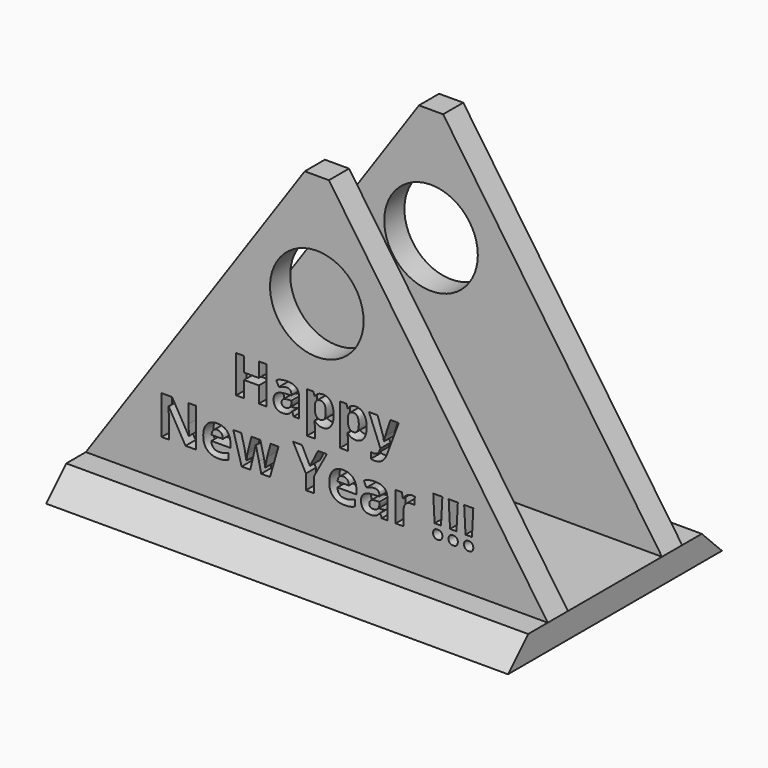
from build123d import *

# Parameters (mm, degrees)
F0_W            = 55
F0_H            = 14
F1_DEPTH        = 3
F2_W            = 55
F2_H            = 3
F3_DEPTH        = 3
F4_W            = 55
F4_H            = 3
F5_DEPTH        = 3
F6_SIZE         = 2.54
F7_W            = 55
F7_H            = 3
F8_DEPTH        = 8
F9_W            = 55
F9_H            = 3
F10_DEPTH       = 8
F11_T1_DEPTH    = 81.1282991577
F12_TEXT_SIZE   = 6.216740762
F12_TEXT_SIZE_2 = 6.4386997967
F13_DEPTH       = 1.5
F14_R           = 5.5706779513
F15_DEPTH       = 25.921


# Not quite as in the source:
# - a fillet or chamfer that OpenCascade refuses, or shapes differently, is made with other operations: its cross-section is extruded or revolved along the edge and cut away or added
# - Text() gives the source's letters only with a copy of the font that has no kerning and outlines rounded to 1/6400 em; it was checked with that copy


with BuildPart() as f1:
    # F0 (on Top) → F1 (new body)
    with BuildSketch(Plane.XY):
        Rectangle(F0_W, F0_H)
    extrude(amount=F1_DEPTH)

    # F2 (on face) → F3 (join)
    with BuildSketch(Plane.XZ.offset(7)):
        with Locations((0, 1.5)):
            Rectangle(F2_W, F2_H)
        Polygon((27.5, 3), (0, 43), (-27.5, 3), align=None)
    extrude(amount=F3_DEPTH)

    # F4 (on face) → F5 (join)
    with BuildSketch(Plane(origin=(0, 7, 0), x_dir=(-1, 0, 0), z_dir=(0, 1, 0))):
        Polygon((0, 43), (-27.5, 3), (27.5, 3), align=None)
        with Locations((0, 1.5)):
            Rectangle(F4_W, F4_H)
    extrude(amount=F5_DEPTH)

    # F6
    f6_edges = [f1.edges().sort_by_distance(p)[0] for p in [
        (0, 8.5, 43),
        (0, -8.5, 43),
    ]]
    chamfer(f6_edges, length=F6_SIZE)

    # F7 (on face) → F8 (join)
    with BuildSketch(Plane.XZ.offset(10)):
        with Locations((0, 1.5)):
            Rectangle(F7_W, F7_H)
    extrude(amount=F8_DEPTH)

    # F9 (on face) → F10 (join)
    with BuildSketch(Plane(origin=(0, 10, 0), x_dir=(-1, 0, 0), z_dir=(0, 1, 0))):
        with Locations((0, 1.5)):
            Rectangle(F9_W, F9_H)
    extrude(amount=F10_DEPTH)

    # F11: chamfer of 5.08 on 2 edges, made by hand

    # F11_s2 → F11_t1 (cut)
    with BuildSketch(Plane.YZ.offset(-40.5641495789)):
        Polygon((18, -2.08), (12.92, 3), (18, 3), align=None)
        Polygon((-12.92, 3), (-18, -2.08), (-18, 3), align=None)
    extrude(amount=F11_T1_DEPTH, mode=Mode.SUBTRACT)

    # F12 (on face) → F13 (cut)
    with BuildSketch(Plane.XZ.offset(10)):
        with Locations((-10.16, 14.7666107269)):
            Text('Happy', F12_TEXT_SIZE, font='Open Sans', font_style=FontStyle.BOLD, text_align=(TextAlign.LEFT, TextAlign.BOTTOM))
        with Locations((-19.05, 7.5160441826)):
            Text('New Year !!!', F12_TEXT_SIZE_2, font='Open Sans', font_style=FontStyle.BOLD, text_align=(TextAlign.LEFT, TextAlign.BOTTOM))
    extrude(amount=-F13_DEPTH, mode=Mode.SUBTRACT)

    # F14 (on face) → F15 (cut, through all)
    with BuildSketch(Plane.XZ.offset(10)):
        with Locations((0, 27.4809952825)):
            Circle(F14_R)
    extrude(amount=-F15_DEPTH, mode=Mode.SUBTRACT)


solid = f1.part
